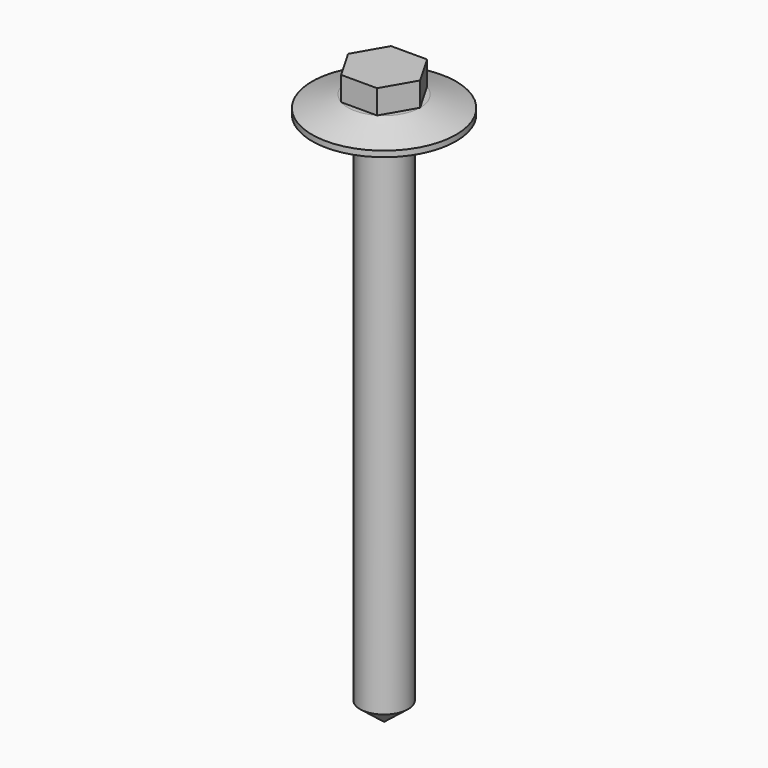
from build123d import *

# Parameters (mm, degrees)
F2_R     = 10.2989039919
F3_DEPTH = 3.175


# Not quite as in the source:
# - a length typed as a fraction of an inch, garbled in the dataset ("3 / 203.2 mm" for 3/8 in), is restored


with BuildPart() as f1:
    # F0 (on Front) → F1 (revolve)
    with BuildSketch(Plane.XZ):
        Polygon((0, 76.2), (0, 0), (3.175, 2.5115670547), (3.175, 70.6755), (9.525, 70.6755), (9.525, 71.4375), (4.7625, 73.025), (4.7625, 76.2), align=None)
    revolve(axis=Axis((0, 0, 38.1), (0, 0, 1)))

    # F2 (on face) → F3 (cut)
    with BuildSketch(Plane.XY.offset(76.2)):
        Circle(F2_R)
        Polygon((-4.7625, 0), (-2.38125, 4.1244459855), (2.38125, 4.1244459855), (4.7625, 0), (2.38125, -4.1244459855), (-2.38125, -4.1244459855), align=None, mode=Mode.SUBTRACT)
    extrude(amount=-F3_DEPTH, mode=Mode.SUBTRACT)


solid = f1.part
